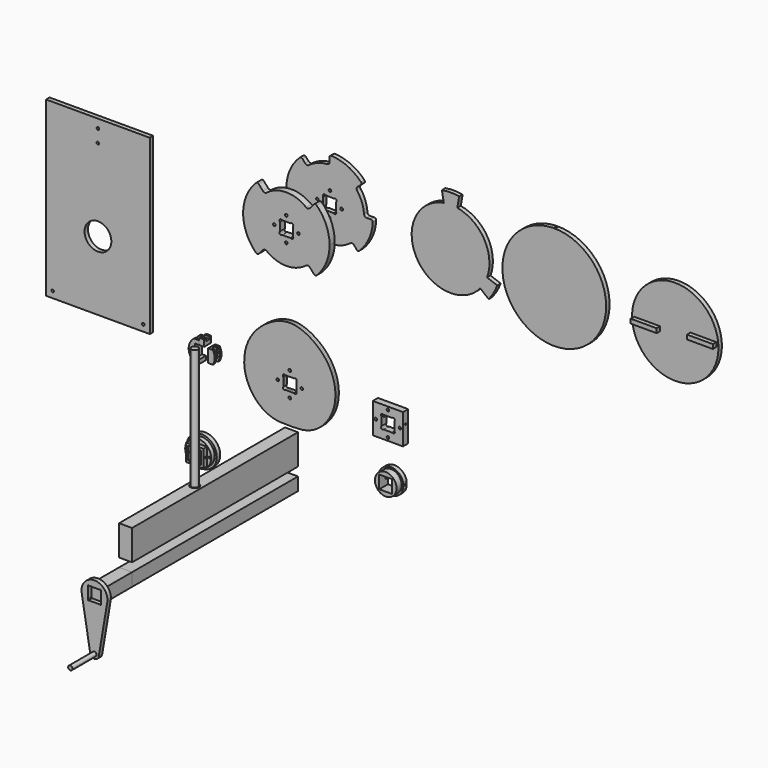
from build123d import *

# Parameters (mm, degrees)
F0_R           = 3.81
F1_DEPTH       = 6.35
F4_DEPTH       = 6.35
F5_START       = 6.35
F5_DEPTH       = 6.35
F7_W           = 304.8
F7_H           = 508
F7_R           = 3.81
F7_R_2         = 39.37
F8_DEPTH       = 12.7
F3_W           = 15.24
F3_H           = 11.7720391928
F9_DEPTH       = 12.7
F10_START      = 6.35
F10_DEPTH      = 6.35
F12_DEPTH      = 12.7
F13_START      = 6.35
F13_DEPTH      = 6.35
F16_W          = 50.8
F16_H          = 50.8
F16_W_2        = 38.1
F16_H_2        = 38.1
F17_DEPTH      = 38.1
F16_R          = 38.1
F16_R_2        = 2.54
F18_DEPTH      = 25.4
F16_R_3        = 44.45
F19_DEPTH      = 12.7
F20_R          = 2.54
F21_DEPTH      = 413.4180533997
F22_W          = 38.1
F22_H          = 38.1
F23_DEPTH      = 711.2
F24_DEPTH      = 609.6
F25_W          = 38.1
F25_H          = 88.9
F26_DEPTH      = 609.6
F27_R          = 12.7
F28_DEPTH      = 88.9
F29_R          = 9.906
F30_DEPTH      = 355.6
F31_R          = 6.35
F32_DEPTH      = 12.7
F33_DEPTH      = 101.6
F34_W          = 88.9
F34_H          = 88.9
F34_R          = 3.81
F35_DEPTH      = 19.05
F36_R          = 2.54
F37_DEPTH      = 88.901
F38_R          = 31.75
F38_W          = 38.1
F38_H          = 38.1
F39_DEPTH      = 19.05
F40_DEPTH      = 12.7
F41_R          = 2.54
F42_DEPTH      = 16.6909680899
F42_DEPTH_BACK = 69.851
F43_R          = 3.81
F44_DEPTH      = 19.05
F45_R          = 5.08
F46_R          = 7.62
F48_R          = 3.81
F49_DEPTH      = 12.7
F50_R          = 5.08
F51_R          = 7.62
F53_DEPTH      = 12.7
F52_R          = 152.4
F54_DEPTH      = 12.7
F55_R          = 127
F55_W          = 76.2
F55_H          = 12.7
F56_DEPTH      = 12.7
F57_DEPTH      = 25.4
F58_R          = 3.2004
F59_DEPTH      = 812.801


with BuildPart() as f1:
    # F0 (on Front) → F1 (new body, symmetric)
    with BuildSketch(Plane.XZ):
        with BuildLine():
            add(Edge.make_bspline(
                [(0, 158.75), (-26.6086433843, 158.75), (-79.0704218132, 134.3104484264), (-128.4996737249, 74.1730285067), (-139.4442596196, -0.6005658595), (-113.0669867076, -65.2785073639), (-60.2927148167, -107.1645221513), (0, -108.3357880752), (60.2927148167, -107.1645221513), (113.0669867076, -65.2785073639), (139.4442596196, -0.6005658595), (128.4996737249, 74.1730285067), (79.0704218132, 134.3104484264), (26.6086433843, 158.75), (0, 158.75)],
                knots=[0, 0, 0, 0, 0.0897830053, 0.177016771, 0.2617339271, 0.3438594583, 0.4233114477, 0.5, 0.5766885523, 0.6561405417, 0.7382660729, 0.822983229, 0.9102169947, 1, 1, 1, 1], degree=3))
        make_face()
        with Locations((-35.56, 0)):
            Circle(F0_R, mode=Mode.SUBTRACT)
        with Locations((0, -35.56)):
            Circle(F0_R, mode=Mode.SUBTRACT)
        with BuildLine():
            Line((12.7, -19.05), (-12.7, -19.05))
            ThreePointArc((-12.7, -19.05), (-19.05, -19.05), (-19.05, -12.7))
            Line((-19.05, -12.7), (-19.05, 12.7))
            ThreePointArc((-19.05, 12.7), (-19.05, 19.05), (-12.7, 19.05))
            Line((-12.7, 19.05), (12.7, 19.05))
            ThreePointArc((12.7, 19.05), (19.05, 19.05), (19.05, 12.7))
            Line((19.05, 12.7), (19.05, -12.7))
            ThreePointArc((19.05, -12.7), (19.05, -19.05), (12.7, -19.05))
        make_face(mode=Mode.SUBTRACT)
        with Locations((35.56, 0)):
            Circle(F0_R, mode=Mode.SUBTRACT)
        with Locations((0, 35.56)):
            Circle(F0_R, mode=Mode.SUBTRACT)
    extrude(amount=F1_DEPTH, both=True)


with BuildPart() as f4:
    # F3 (on Front) → F4 (new body)
    with BuildSketch(Plane.XZ):
        with BuildLine():
            Line((-261.62, 19.05), (-261.62, 30.8220391928))
            ThreePointArc((-261.62, 30.8220391928), (-285.75, 0), (-261.62, -30.8220391928))
            Line((-261.62, -30.8220391928), (-261.62, -19.05))
            Line((-261.62, -19.05), (-273.05, -19.05))
            Line((-273.05, -19.05), (-273.05, 19.05))
            Line((-273.05, 19.05), (-261.62, 19.05))
        make_face()
    extrude(amount=F4_DEPTH)

    # F3 (on Front) → F5 (join)
    with BuildSketch(Plane.XZ.offset(F5_START)):
        with BuildLine():
            ThreePointArc((-261.62, -30.8220391928), (-285.75, 0), (-261.62, 30.8220391928))
            Line((-261.62, 30.8220391928), (-276.3966939525, 30.8220391928))
            ThreePointArc((-276.3966939525, 30.8220391928), (-292.1, 0), (-276.3966939525, -30.8220391928))
            Line((-276.3966939525, -30.8220391928), (-261.62, -30.8220391928))
        make_face()
        with BuildLine():
            Line((-261.62, 19.05), (-261.62, 30.8220391928))
            ThreePointArc((-261.62, 30.8220391928), (-285.75, 0), (-261.62, -30.8220391928))
            Line((-261.62, -30.8220391928), (-261.62, -19.05))
            Line((-261.62, -19.05), (-273.05, -19.05))
            Line((-273.05, -19.05), (-273.05, 19.05))
            Line((-273.05, 19.05), (-261.62, 19.05))
        make_face()
    extrude(amount=F5_DEPTH)

    # F6: F4 across plane


with BuildPart() as f4_1:
    add(f4.part)
    add(f4.part.mirror(Plane.XZ))


with BuildPart() as f8:
    # F7 (on Front) → F8 (new body)
    with BuildSketch(Plane.XZ):
        with Locations((-558.8, 254)):
            Rectangle(F7_W, F7_H)
        with Locations((-692.15, 19.05)):
            Circle(F7_R, mode=Mode.SUBTRACT)
        with Locations((-425.45, 19.05)):
            Circle(F7_R, mode=Mode.SUBTRACT)
        with Locations((-558.8, 203.2)):
            Circle(F7_R_2, mode=Mode.SUBTRACT)
        with Locations((-558.8, 444.5)):
            Circle(F7_R, mode=Mode.SUBTRACT)
        with Locations((-558.8, 482.6)):
            Circle(F7_R, mode=Mode.SUBTRACT)
    extrude(amount=F8_DEPTH)


with BuildPart() as f9:
    # F3 (on Front) → F9 (new body)
    with BuildSketch(Plane.XZ):
        with Locations((-254, 24.9360195964)):
            Rectangle(F3_W, F3_H)
        with BuildLine():
            Line((-261.62, 30.8220391928), (-246.38, 30.8220391928))
            ThreePointArc((-246.38, 30.8220391928), (-254, 31.75), (-261.62, 30.8220391928))
        make_face()
    extrude(amount=F9_DEPTH)

    # F3 (on Front) → F10 (join)
    with BuildSketch(Plane.XZ.offset(F10_START)):
        with BuildLine():
            Line((-246.38, 30.8220391928), (-246.38, 37.33022368))
            ThreePointArc((-246.38, 37.33022368), (-254, 38.1), (-261.62, 37.33022368))
            Line((-261.62, 37.33022368), (-261.62, 30.8220391928))
            ThreePointArc((-261.62, 30.8220391928), (-254, 31.75), (-246.38, 30.8220391928))
        make_face()
    extrude(amount=F10_DEPTH)

    # F11: F9 across plane


with BuildPart() as f9_1:
    add(f9.part)
    add(f9.part.mirror(Plane.XZ))


with BuildPart() as f12:
    # F3 (on Front) → F12 (new body)
    with BuildSketch(Plane.XZ):
        with BuildLine():
            ThreePointArc((-222.25, 0), (-223.8793052869, 10.040231571), (-228.6, 19.05))
            Line((-228.6, 19.05), (-234.95, 19.05))
            Line((-234.95, 19.05), (-234.95, -19.05))
            Line((-234.95, -19.05), (-228.6, -19.05))
            ThreePointArc((-228.6, -19.05), (-223.8793052869, -10.040231571), (-222.25, 0))
        make_face()
    extrude(amount=F12_DEPTH)

    # F3 (on Front) → F13 (join)
    with BuildSketch(Plane.XZ.offset(F13_START)):
        with BuildLine():
            ThreePointArc((-221.0044321158, -19.05), (-217.1982260184, -9.8610056184), (-215.9, 0))
            ThreePointArc((-215.9, 0), (-217.1982260184, 9.8610056184), (-221.0044321158, 19.05))
            Line((-221.0044321158, 19.05), (-228.6, 19.05))
            ThreePointArc((-228.6, 19.05), (-223.8793052869, 10.040231571), (-222.25, 0))
            ThreePointArc((-222.25, 0), (-223.8793052869, -10.040231571), (-228.6, -19.05))
            Line((-228.6, -19.05), (-221.0044321158, -19.05))
        make_face()
    extrude(amount=F13_DEPTH)

    # F14: F12 across plane


with BuildPart() as f12_1:
    add(f12.part)
    add(f12.part.mirror(Plane.XZ))


with BuildPart() as f17:
    # F16 (on Front) → F17 (new body)
    with BuildSketch(Plane.XZ):
        with Locations((-254, -254)):
            Rectangle(F16_W, F16_H)
        with Locations((-254, -254)):
            Rectangle(F16_W_2, F16_H_2, mode=Mode.SUBTRACT)
    extrude(amount=F17_DEPTH)

    # F16 (on Front) → F18 (join)
    with BuildSketch(Plane.XZ):
        with Locations((-254, -254)):
            Circle(F16_R)
        with Locations((-254, -287.02)):
            Circle(F16_R_2, mode=Mode.SUBTRACT)
        with Locations((-287.02, -254)):
            Circle(F16_R_2, mode=Mode.SUBTRACT)
        with Locations((-254, -254)):
            Rectangle(F16_W, F16_H, mode=Mode.SUBTRACT)
        with Locations((-220.98, -254)):
            Circle(F16_R_2, mode=Mode.SUBTRACT)
        with Locations((-254, -220.98)):
            Circle(F16_R_2, mode=Mode.SUBTRACT)
    extrude(amount=F18_DEPTH)

    # F16 (on Front) → F19 (join)
    with BuildSketch(Plane.XZ):
        with Locations((-254, -254)):
            Circle(F16_R_3)
        with Locations((-254, -254)):
            Circle(F16_R, mode=Mode.SUBTRACT)
    extrude(amount=F19_DEPTH)

    # F20 (on face) → F21 (cut, through all)
    with BuildSketch(Plane(origin=(-279.4, 0, 0), x_dir=(0, -1, 0), z_dir=(-1, 0, 0))):
        with Locations((31.75, -254)):
            Circle(F20_R)
    extrude(amount=-F21_DEPTH, mode=Mode.SUBTRACT)


with BuildPart() as f23:
    # F22 (on Front) → F23 (new body)
    with BuildSketch(Plane.XZ):
        with Locations((0, -254)):
            Rectangle(F22_W, F22_H)
    extrude(amount=F23_DEPTH)


with BuildPart() as f24:
    # F22 (on Front) → F24 (new body)
    with BuildSketch(Plane.XZ):
        with Locations((0, -254)):
            Rectangle(F22_W, F22_H)
    extrude(amount=F24_DEPTH)


with BuildPart() as f26:
    # F25 (on Front) → F26 (new body)
    with BuildSketch(Plane.XZ):
        with Locations((0, -165.1)):
            Rectangle(F25_W, F25_H)
    extrude(amount=F26_DEPTH)

    # F27 (on face) → F28 (cut, through all)
    with BuildSketch(Plane.XY.offset(-120.65)):
        with Locations((0, -355.6)):
            Circle(F27_R)
    extrude(amount=-F28_DEPTH, mode=Mode.SUBTRACT)


with BuildPart() as f30:
    # F29 (on face) → F30 (new body)
    with BuildSketch(Plane.XY.offset(-120.65)):
        with Locations((0, -355.6)):
            Circle(F29_R)
    extrude(amount=F30_DEPTH)


with BuildPart() as f32:
    # F31 (on face) → F32 (new body)
    with BuildSketch(Plane.XZ.offset(711.2)):
        with BuildLine():
            ThreePointArc((37.5671066227, -260.35), (0, -292.1), (-37.5671066227, -260.35))
            Line((-37.5671066227, -260.35), (-12.5223688742, -408.5166666667))
            ThreePointArc((-12.5223688742, -408.5166666667), (-1.0620535056, -393.7444856939), (12.7, -406.4))
            ThreePointArc((12.7, -406.4), (12.6555143061, -407.4620535056), (12.5223688742, -408.5166666667))
            Line((12.5223688742, -408.5166666667), (37.5671066227, -260.35))
        make_face()
        with BuildLine():
            ThreePointArc((12.7, -406.4), (-1.0620535056, -393.7444856939), (-12.5223688742, -408.5166666667))
            ThreePointArc((-12.5223688742, -408.5166666667), (0, -419.1), (12.5223688742, -408.5166666667))
            ThreePointArc((12.5223688742, -408.5166666667), (12.6555143061, -407.4620535056), (12.7, -406.4))
        make_face()
        with Locations((0, -406.4)):
            Circle(F31_R, mode=Mode.SUBTRACT)
        with BuildLine():
            ThreePointArc((37.5671066227, -260.35), (37.9665429182, -257.1861605167), (38.1, -254))
            ThreePointArc((38.1, -254), (-3.1861605167, -216.0334570818), (-37.5671066227, -260.35))
            ThreePointArc((-37.5671066227, -260.35), (0, -292.1), (37.5671066227, -260.35))
        make_face()
        with BuildLine():
            ThreePointArc((-19.05, -234.95), (-17.4625, -234.2924359697), (-15.875, -234.95))
            Line((-15.875, -234.95), (15.875, -234.95))
            ThreePointArc((15.875, -234.95), (17.4625, -234.2924359697), (19.05, -234.95))
            ThreePointArc((19.05, -234.95), (19.7075640303, -236.5375), (19.05, -238.125))
            Line((19.05, -238.125), (19.05, -269.875))
            ThreePointArc((19.05, -269.875), (19.7075640303, -271.4625), (19.05, -273.05))
            ThreePointArc((19.05, -273.05), (17.4625, -273.7075640303), (15.875, -273.05))
            Line((15.875, -273.05), (-15.875, -273.05))
            ThreePointArc((-15.875, -273.05), (-17.4625, -273.7075640303), (-19.05, -273.05))
            ThreePointArc((-19.05, -273.05), (-19.7075640303, -271.4625), (-19.05, -269.875))
            Line((-19.05, -269.875), (-19.05, -238.125))
            ThreePointArc((-19.05, -238.125), (-19.7075640303, -236.5375), (-19.05, -234.95))
        make_face(mode=Mode.SUBTRACT)
    extrude(amount=F32_DEPTH)

    # F31 (on face) → F33 (join)
    with BuildSketch(Plane.XZ.offset(711.2)):
        with Locations((0, -406.4)):
            Circle(F31_R)
    extrude(amount=F33_DEPTH)


with BuildPart() as f35:
    # F34 (on Front) → F35 (new body)
    with BuildSketch(Plane.XZ):
        with Locations((298.45, 0)):
            Rectangle(F34_W, F34_H)
        with Locations((298.45, -35.56)):
            Circle(F34_R, mode=Mode.SUBTRACT)
        with Locations((262.89, 0)):
            Circle(F34_R, mode=Mode.SUBTRACT)
        with BuildLine():
            ThreePointArc((279.4, 12.7), (278.0848719395, 15.875), (279.4, 19.05))
            ThreePointArc((279.4, 19.05), (282.575, 20.3651280605), (285.75, 19.05))
            Line((285.75, 19.05), (311.15, 19.05))
            ThreePointArc((311.15, 19.05), (314.325, 20.3651280605), (317.5, 19.05))
            ThreePointArc((317.5, 19.05), (318.4733374135, 17.593297618), (318.8151280605, 15.875))
            ThreePointArc((318.8151280605, 15.875), (318.4733374135, 14.156702382), (317.5, 12.7))
            Line((317.5, 12.7), (317.5, -12.7))
            ThreePointArc((317.5, -12.7), (318.4733374135, -14.156702382), (318.8151280605, -15.875))
            ThreePointArc((318.8151280605, -15.875), (318.4733374135, -17.593297618), (317.5, -19.05))
            ThreePointArc((317.5, -19.05), (314.325, -20.3651280605), (311.15, -19.05))
            Line((311.15, -19.05), (285.75, -19.05))
            ThreePointArc((285.75, -19.05), (282.575, -20.3651280605), (279.4, -19.05))
            ThreePointArc((279.4, -19.05), (278.0848719395, -15.875), (279.4, -12.7))
            Line((279.4, -12.7), (279.4, 12.7))
        make_face(mode=Mode.SUBTRACT)
        with Locations((334.01, 0)):
            Circle(F34_R, mode=Mode.SUBTRACT)
        with Locations((298.45, 35.56)):
            Circle(F34_R, mode=Mode.SUBTRACT)
    extrude(amount=F35_DEPTH)

    # F36 (on face) → F37 (cut, through all)
    with BuildSketch(Plane(origin=(254, 0, 0), x_dir=(0, -1, 0), z_dir=(-1, 0, 0))):
        with Locations((9.525, 9.525)):
            Circle(F36_R)
    extrude(amount=-F37_DEPTH, mode=Mode.SUBTRACT)


with BuildPart() as f39:
    # F38 (on Front) → F39 (new body)
    with BuildSketch(Plane.XZ):
        with Locations((292.1, -158.75)):
            Circle(F38_R)
        with Locations((292.1, -158.75)):
            Rectangle(F38_W, F38_H, mode=Mode.SUBTRACT)
    extrude(amount=F39_DEPTH)

    # F38 (on Front) → F40 (join)
    with BuildSketch(Plane.XZ):
        with BuildLine():
            Line((327.8409680899, -167.64), (327.8409680899, -149.86))
            ThreePointArc((327.8409680899, -149.86), (292.1, -121.92), (256.3590319101, -149.86))
            Line((256.3590319101, -149.86), (256.3590319101, -167.64))
            ThreePointArc((256.3590319101, -167.64), (292.1, -195.58), (327.8409680899, -167.64))
        make_face()
        with Locations((292.1, -158.75)):
            Circle(F38_R, mode=Mode.SUBTRACT)
        with Locations((292.1, -158.75)):
            Circle(F38_R)
        with Locations((292.1, -158.75)):
            Rectangle(F38_W, F38_H, mode=Mode.SUBTRACT)
    extrude(amount=-F40_DEPTH)

    # F41 (on face) → F42 (cut, two sides)
    with BuildSketch(Plane.YZ.offset(273.05)) as f42_sk:
        with Locations((6.35, -158.75)):
            Circle(F41_R)
    extrude(amount=-F42_DEPTH, mode=Mode.SUBTRACT)
    extrude(f42_sk.sketch, amount=F42_DEPTH_BACK, mode=Mode.SUBTRACT)


with BuildPart() as f44:
    # F43 (on Front) → F44 (new body)
    with BuildSketch(Plane.XZ):
        with BuildLine():
            ThreePointArc((95.25, 406.4), (87.0152048405, 445.141665253), (63.7346902557, 477.1845446267))
            ThreePointArc((63.7346902557, 477.1845446267), (0, 501.65), (-63.7346902557, 477.1845446267))
            ThreePointArc((-63.7346902557, 477.1845446267), (-95.25, 406.4), (-63.7346902557, 335.6154553733))
            ThreePointArc((-63.7346902557, 335.6154553733), (0, 311.15), (63.7346902557, 335.6154553733))
            ThreePointArc((63.7346902557, 335.6154553733), (87.0152048405, 367.658334747), (95.25, 406.4))
        make_face()
        with Locations((0, 370.84)):
            Circle(F43_R, mode=Mode.SUBTRACT)
        with Locations((-35.56, 406.4)):
            Circle(F43_R, mode=Mode.SUBTRACT)
        with BuildLine():
            ThreePointArc((-19.05, 419.1), (-20.3651280605, 422.275), (-19.05, 425.45))
            ThreePointArc((-19.05, 425.45), (-15.875, 426.7651280605), (-12.7, 425.45))
            Line((-12.7, 425.45), (12.7, 425.45))
            ThreePointArc((12.7, 425.45), (15.875, 426.7651280605), (19.05, 425.45))
            ThreePointArc((19.05, 425.45), (20.0233374135, 423.993297618), (20.3651280605, 422.275))
            ThreePointArc((20.3651280605, 422.275), (20.0233374135, 420.556702382), (19.05, 419.1))
            Line((19.05, 419.1), (19.05, 393.7))
            ThreePointArc((19.05, 393.7), (20.0233374135, 392.243297618), (20.3651280605, 390.525))
            ThreePointArc((20.3651280605, 390.525), (20.0233374135, 388.806702382), (19.05, 387.35))
            ThreePointArc((19.05, 387.35), (15.875, 386.0348719395), (12.7, 387.35))
            Line((12.7, 387.35), (-12.7, 387.35))
            ThreePointArc((-12.7, 387.35), (-15.875, 386.0348719395), (-19.05, 387.35))
            ThreePointArc((-19.05, 387.35), (-20.3651280605, 390.525), (-19.05, 393.7))
            Line((-19.05, 393.7), (-19.05, 419.1))
        make_face(mode=Mode.SUBTRACT)
        with Locations((35.56, 406.4)):
            Circle(F43_R, mode=Mode.SUBTRACT)
        with Locations((0, 441.96)):
            Circle(F43_R, mode=Mode.SUBTRACT)
        with BuildLine():
            Line((-63.7346902557, 477.1845446267), (-84.9795870076, 500.7793928356))
            ThreePointArc((-84.9795870076, 500.7793928356), (-127, 406.4), (-84.9795870076, 312.0206071644))
            Line((-84.9795870076, 312.0206071644), (-63.7346902557, 335.6154553733))
            ThreePointArc((-63.7346902557, 335.6154553733), (-95.25, 406.4), (-63.7346902557, 477.1845446267))
        make_face()
        with BuildLine():
            ThreePointArc((84.9795870076, 312.0206071644), (116.0202731206, 354.7444463294), (127, 406.4))
            ThreePointArc((127, 406.4), (116.0202731206, 458.0555536706), (84.9795870076, 500.7793928356))
            Line((84.9795870076, 500.7793928356), (63.7346902557, 477.1845446267))
            ThreePointArc((63.7346902557, 477.1845446267), (87.0152048405, 445.141665253), (95.25, 406.4))
            ThreePointArc((95.25, 406.4), (87.0152048405, 367.658334747), (63.7346902557, 335.6154553733))
            Line((63.7346902557, 335.6154553733), (84.9795870076, 312.0206071644))
        make_face()
    extrude(amount=F44_DEPTH)

    # F45
    f45_edges = [f44.edges().sort_by_distance(p)[0] for p in [
        (-84.979587, -9.525, 500.779393),
        (84.979587, -9.525, 500.779393),
        (84.979587, -9.525, 312.020607),
        (-84.979587, -9.525, 312.020607),
    ]]
    fillet(f45_edges, radius=F45_R)

    # F46
    f46_edges = [f44.edges().sort_by_distance(p)[0] for p in [
        (-63.73469, -9.525, 477.184545),
        (63.73469, -9.525, 477.184545),
        (-63.73469, -9.525, 335.615455),
        (63.73469, -9.525, 335.615455),
    ]]
    fillet(f46_edges, radius=F46_R)


with BuildPart() as f49:
    # F48 (on offset) → F49 (new body)
    with BuildSketch(Plane.XZ.offset(-152.4)):
        with BuildLine():
            Line((-66.6555973454, 483.0784933506), (-83.3194966818, 502.2481166883))
            ThreePointArc((-83.3194966818, 502.2481166883), (-115.5650814013, 459.0660418173), (-127, 406.4))
            Line((-127, 406.4), (-101.6, 406.4))
            ThreePointArc((-101.6, 406.4), (-95.1658944276, 370.818930064), (-76.6784933506, 339.7444026546))
            Line((-76.6784933506, 339.7444026546), (-95.8481166883, 323.0805033182))
            ThreePointArc((-95.8481166883, 323.0805033182), (-52.6660418173, 290.8349185987), (0, 279.4))
            Line((0, 279.4), (0, 304.8))
            ThreePointArc((0, 304.8), (35.581069936, 311.2341055724), (66.6555973454, 329.7215066494))
            Line((66.6555973454, 329.7215066494), (83.3194966818, 310.5518833117))
            ThreePointArc((83.3194966818, 310.5518833117), (115.5650814013, 353.7339581827), (127, 406.4))
            Line((127, 406.4), (101.6, 406.4))
            ThreePointArc((101.6, 406.4), (95.1658944276, 441.981069936), (76.6784933506, 473.0555973454))
            Line((76.6784933506, 473.0555973454), (95.8481166883, 489.7194966818))
            ThreePointArc((95.8481166883, 489.7194966818), (52.6660418173, 521.9650814013), (0, 533.4))
            Line((0, 533.4), (0, 508))
            ThreePointArc((0, 508), (-35.581069936, 501.5658944276), (-66.6555973454, 483.0784933506))
        make_face()
        with Locations((-1.2417825631, 370.84)):
            Circle(F48_R, mode=Mode.SUBTRACT)
        with Locations((35.56, 405.1582174369)):
            Circle(F48_R, mode=Mode.SUBTRACT)
        with Locations((-35.56, 407.6417825631)):
            Circle(F48_R, mode=Mode.SUBTRACT)
        with BuildLine():
            ThreePointArc((-18.5951716466, 419.7570989153), (-19.7986926646, 422.9760620985), (-18.3735598425, 426.1032306669))
            ThreePointArc((-18.3735598425, 426.1032306669), (-15.1545966593, 427.3067516849), (-12.027428091, 425.8816188628))
            Line((-12.027428091, 425.8816188628), (13.3570989153, 424.9951716466))
            ThreePointArc((13.3570989153, 424.9951716466), (16.5760620985, 426.1986926646), (19.7032306669, 424.7735598425))
            ThreePointArc((19.7032306669, 424.7735598425), (20.5970529191, 423.3569373111), (20.9094869496, 421.7112998688))
            ThreePointArc((20.9094869496, 421.7112998688), (20.5370760623, 419.9208654853), (19.4816188628, 418.427428091))
            Line((19.4816188628, 418.427428091), (18.5951716466, 393.0429010847))
            ThreePointArc((18.5951716466, 393.0429010847), (19.4889938988, 391.6262785533), (19.8014279293, 389.9806411109))
            ThreePointArc((19.8014279293, 389.9806411109), (19.429017042, 388.1902067274), (18.3735598425, 386.6967693331))
            ThreePointArc((18.3735598425, 386.6967693331), (15.1545966593, 385.4932483151), (12.027428091, 386.9183811372))
            Line((12.027428091, 386.9183811372), (-13.3570989153, 387.8048283534))
            ThreePointArc((-13.3570989153, 387.8048283534), (-16.5760620985, 386.6013073354), (-19.7032306669, 388.0264401575))
            ThreePointArc((-19.7032306669, 388.0264401575), (-20.9067516849, 391.2454033407), (-19.4816188628, 394.372571909))
            Line((-19.4816188628, 394.372571909), (-18.5951716466, 419.7570989153))
        make_face(mode=Mode.SUBTRACT)
        with Locations((1.2417825631, 441.96)):
            Circle(F48_R, mode=Mode.SUBTRACT)
    extrude(amount=F49_DEPTH)

    # F50
    f50_edges = [f49.edges().sort_by_distance(p)[0] for p in [
        (95.848117, 146.05, 489.719497),
        (127, 146.05, 406.4),
        (83.319497, 146.05, 310.551883),
        (0, 146.05, 279.4),
        (-95.848117, 146.05, 323.080503),
        (-127, 146.05, 406.4),
        (-83.319497, 146.05, 502.248117),
        (0, 146.05, 533.4),
    ]]
    fillet(f50_edges, radius=F50_R)

    # F51
    f51_edges = [f49.edges().sort_by_distance(p)[0] for p in [
        (0, 146.05, 508),
        (76.678493, 146.05, 473.055597),
        (101.6, 146.05, 406.4),
        (66.655597, 146.05, 329.721507),
        (0, 146.05, 304.8),
        (-76.678493, 146.05, 339.744403),
        (-101.6, 146.05, 406.4),
        (-66.655597, 146.05, 483.078493),
    ]]
    fillet(f51_edges, radius=F51_R)


with BuildPart() as f53:
    # F52 (on offset) → F53 (new body)
    with BuildSketch(Plane.XZ.offset(-152.4)):
        with BuildLine():
            Line((330.2386836517, 550.2311723274), (335.7520132927, 518.9635261693))
            ThreePointArc((335.7520132927, 518.9635261693), (256.6132963474, 349.25), (443.1588798485, 332.9293762128))
            Line((443.1588798485, 332.9293762128), (467.4807909175, 312.5208696053))
            ThreePointArc((467.4807909175, 312.5208696053), (482.0830102227, 333.375), (492.8421072658, 356.4479580673))
            Line((492.8421072658, 356.4479580673), (463.0068665558, 367.3070976179))
            ThreePointArc((463.0068665558, 367.3070976179), (454.5867036526, 463.55), (375.4479867073, 518.9635261693))
            Line((375.4479867073, 518.9635261693), (380.9613163483, 550.2311723274))
            ThreePointArc((380.9613163483, 550.2311723274), (355.6, 552.45), (330.2386836517, 550.2311723274))
        make_face()
    extrude(amount=F53_DEPTH)


with BuildPart() as f54:
    # F52 (on offset) → F54 (new body)
    with BuildSketch(Plane.XZ.offset(-152.4)):
        with Locations((660.4, 406.4)):
            Circle(F52_R)
    extrude(amount=F54_DEPTH)

    # F58 (on offset) → F59 (cut, through all)
    with BuildSketch(Plane.XY.offset(-254)):
        with Locations((660.4, 146.05)):
            Circle(F58_R)
    extrude(amount=F59_DEPTH, mode=Mode.SUBTRACT)


with BuildPart() as f56:
    # F55 (on offset) → F56 (new body)
    with BuildSketch(Plane.XZ.offset(-152.4)):
        with Locations((1016, 406.4)):
            Circle(F55_R)
        with Locations((933.45, 400.05)):
            Rectangle(F55_W, F55_H, mode=Mode.SUBTRACT)
        with Locations((1098.55, 412.75)):
            Rectangle(F55_W, F55_H, mode=Mode.SUBTRACT)
    extrude(amount=F56_DEPTH)

    # F55 (on offset) → F57 (join)
    with BuildSketch(Plane.XZ.offset(-152.4)):
        with Locations((933.45, 400.05)):
            Rectangle(F55_W, F55_H)
        with Locations((1098.55, 412.75)):
            Rectangle(F55_W, F55_H)
    extrude(amount=F57_DEPTH)


solid = Compound([f1.part, f4_1.part, f8.part, f9_1.part, f12_1.part, f17.part, f23.part, f24.part, f26.part, f30.part, f32.part, f35.part, f39.part, f44.part, f49.part, f53.part, f54.part, f56.part])
